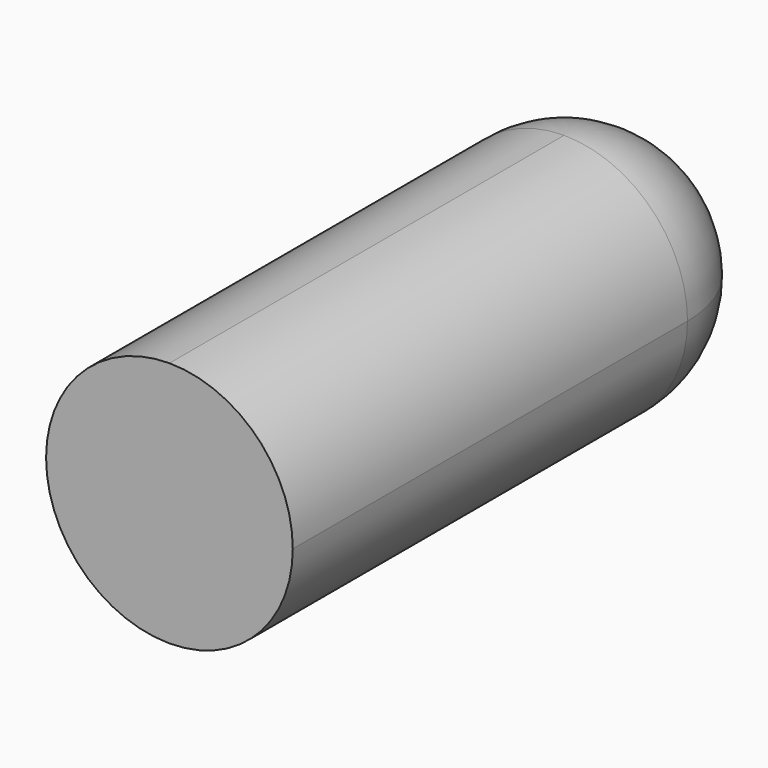
from build123d import *

# Parameters (mm, degrees)
F1_DEPTH = 60
F2_R     = 29.99999


# Not quite as in the source:
# - a fillet or chamfer is up to 0.001 mm smaller than in the source, because OpenCascade refuses the exact size


with BuildPart() as f1:
    # F0 (on Top) → F1 (new body)
    with BuildSketch(Plane.XY):
        with BuildLine():
            ThreePointArc((-10.2322225652, 35.2245123306), (-31.4454260008, 26.4377157662), (-40.2322225652, 5.2245123306))
            Line((-40.2322225652, 5.2245123306), (-40.2322225652, -114.7754876694))
            Line((-40.2322225652, -114.7754876694), (19.7677774348, -114.7754876694))
            Line((19.7677774348, -114.7754876694), (19.7677774348, 5.2245123306))
            ThreePointArc((19.7677774348, 5.2245123306), (10.9809808704, 26.4377157662), (-10.2322225652, 35.2245123306))
        make_face()
    extrude(amount=F1_DEPTH)

    # F2 (radius 30 in the source; OpenCascade refuses exactly that, so slightly less here)
    f2_edges = [f1.edges().sort_by_distance(p)[0] for p in [
        (-40.232223, -54.775488, 0),
        (-40.232223, -54.775488, 60),
    ]]
    fillet(f2_edges, radius=F2_R)


solid = f1.part
